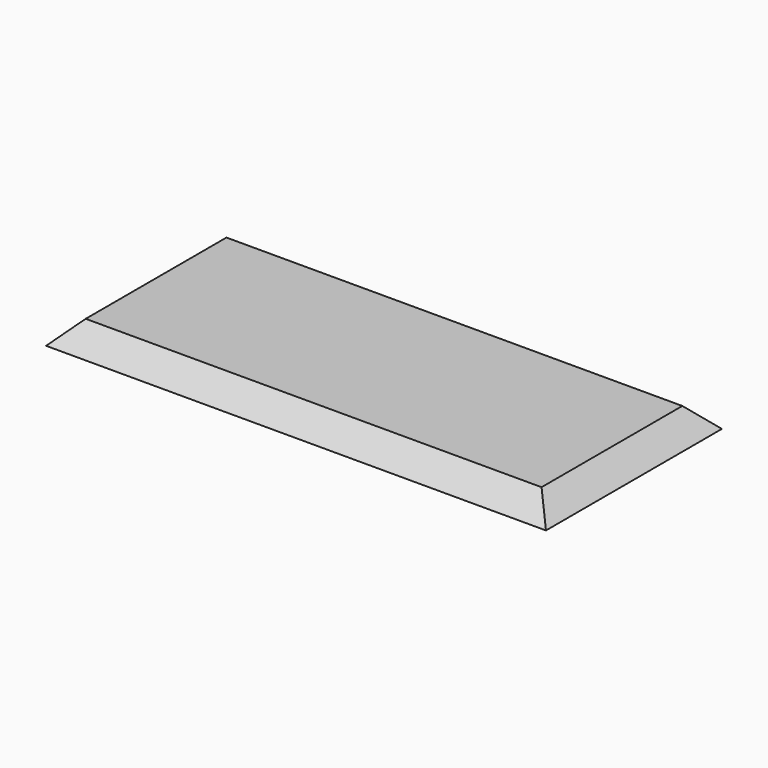
from build123d import *

# Parameters (mm, degrees)
F0_W     = 500
F0_H     = 220
F1_DEPTH = 22
F2_SIZE  = 21.99999


# Not quite as in the source:
# - a fillet or chamfer is up to 0.001 mm smaller than in the source, because OpenCascade refuses the exact size


with BuildPart() as f1:
    # F0 (on Top) → F1 (new body)
    with BuildSketch(Plane.XY):
        Rectangle(F0_W, F0_H)
    extrude(amount=F1_DEPTH)

    # F2 (size 22 in the source; OpenCascade refuses exactly that, so slightly less here)
    f2_edges = [f1.edges().sort_by_distance(p)[0] for p in [
        (250, 0, 22),
        (0, -110, 22),
        (-250, 0, 22),
        (0, 110, 22),
    ]]
    chamfer(f2_edges, length=F2_SIZE)


solid = f1.part
